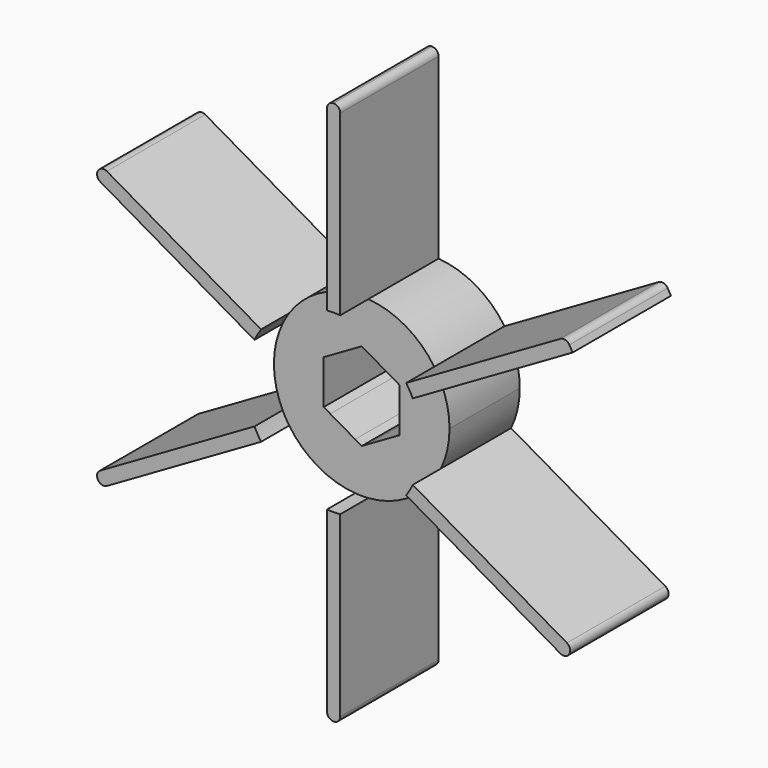
from build123d import *

# Parameters (mm, degrees)
F1_DEPTH = 10
F2_DEPTH = 14
F3_R     = 0.74999


# Not quite as in the source:
# - a fillet or chamfer is up to 0.001 mm smaller than in the source, because OpenCascade refuses the exact size
# - a feature names something its author has since deleted; it is built from what else it names


with BuildPart() as f1:
    # F0 (on Front) → F1 (new body)
    with BuildSketch(Plane.XZ):
        with BuildLine():
            ThreePointArc((9.0108627247, -4.336398616), (9.7495801768, -2.22388992), (10, 0))
            ThreePointArc((10, 0), (9.7495801768, 2.22388992), (9.0108627247, 4.336398616))
            Line((9.0108627247, 4.336398616), (4.6561359474, 1.8221959388))
            ThreePointArc((4.6561359474, 1.8221959388), (4.9132819854, 0.9271785866), (5, 0))
            ThreePointArc((5, 0), (4.9132819854, -0.9271785866), (4.6561359474, -1.8221959388))
            Line((4.6561359474, -1.8221959388), (9.0108627247, -4.336398616))
        make_face()
        with BuildLine():
            Line((4.6561359474, 1.8221959388), (9.0108627247, 4.336398616))
            ThreePointArc((9.0108627247, 4.336398616), (8.6602540378, 5), (8.2608627247, 5.6354367216))
            Line((8.2608627247, 5.6354367216), (3.9061359474, 3.1212340445))
            ThreePointArc((3.9061359474, 3.1212340445), (4.1298292758, 2.8186007438), (4.3301270189, 2.5))
            ThreePointArc((4.3301270189, 2.5), (4.5058944851, 2.1672366942), (4.6561359474, 1.8221959388))
        make_face()
        with BuildLine():
            ThreePointArc((8.2608627247, -5.6354367216), (8.6602540378, -5), (9.0108627247, -4.336398616))
            Line((9.0108627247, -4.336398616), (4.6561359474, -1.8221959388))
            ThreePointArc((4.6561359474, -1.8221959388), (4.5058944851, -2.1672366942), (4.3301270189, -2.5))
            ThreePointArc((4.3301270189, -2.5), (4.1298292758, -2.8186007438), (3.9061359474, -3.1212340445))
            Line((3.9061359474, -3.1212340445), (8.2608627247, -5.6354367216))
        make_face()
        with BuildLine():
            Line((3.9061359474, 3.1212340445), (8.2608627247, 5.6354367216))
            ThreePointArc((8.2608627247, 5.6354367216), (5, 8.6602540378), (0.75, 9.9718353376))
            Line((0.75, 9.9718353376), (0.75, 4.9434299833))
            ThreePointArc((0.75, 4.9434299833), (2.5, 4.3301270189), (3.9061359474, 3.1212340445))
        make_face()
        with BuildLine():
            Line((4.3301270189, 1.6339745962), (4.6561359474, 1.8221959388))
            ThreePointArc((4.6561359474, 1.8221959388), (4.5058944851, 2.1672366942), (4.3301270189, 2.5))
            Line((4.3301270189, 2.5), (4.3301270189, 1.6339745962))
        make_face()
        with BuildLine():
            ThreePointArc((5, 0), (4.9132819854, 0.9271785866), (4.6561359474, 1.8221959388))
            Line((4.6561359474, 1.8221959388), (4.3301270189, 1.6339745962))
            Line((4.3301270189, 1.6339745962), (4.3301270189, -1.6339745962))
            Line((4.3301270189, -1.6339745962), (4.6561359474, -1.8221959388))
            ThreePointArc((4.6561359474, -1.8221959388), (4.9132819854, -0.9271785866), (5, 0))
        make_face()
        with BuildLine():
            ThreePointArc((0.75, -9.9718353376), (5, -8.6602540378), (8.2608627247, -5.6354367216))
            Line((8.2608627247, -5.6354367216), (3.9061359474, -3.1212340445))
            ThreePointArc((3.9061359474, -3.1212340445), (2.5, -4.3301270189), (0.75, -4.9434299833))
            Line((0.75, -4.9434299833), (0.75, -9.9718353376))
        make_face()
        with BuildLine():
            ThreePointArc((4.3301270189, -2.5), (4.5058944851, -2.1672366942), (4.6561359474, -1.8221959388))
            Line((4.6561359474, -1.8221959388), (4.3301270189, -1.6339745962))
            Line((4.3301270189, -1.6339745962), (4.3301270189, -2.5))
        make_face()
        with BuildLine():
            Line((0.75, 4.9434299833), (0.75, 9.9718353376))
            ThreePointArc((0.75, 9.9718353376), (0, 10), (-0.75, 9.9718353376))
            Line((-0.75, 9.9718353376), (-0.75, 4.9434299833))
            ThreePointArc((-0.75, 4.9434299833), (-0.3760652094, 4.985837438), (0, 5))
            ThreePointArc((0, 5), (0.3760652094, 4.985837438), (0.75, 4.9434299833))
        make_face()
        with BuildLine():
            Line((3.5801270189, 2.9330127019), (3.9061359474, 3.1212340445))
            ThreePointArc((3.9061359474, 3.1212340445), (2.5, 4.3301270189), (0.75, 4.9434299833))
            Line((0.75, 4.9434299833), (0.75, 4.5669872981))
            Line((0.75, 4.5669872981), (3.5801270189, 2.9330127019))
        make_face()
        with BuildLine():
            ThreePointArc((4.3301270189, 2.5), (4.1298292758, 2.8186007438), (3.9061359474, 3.1212340445))
            Line((3.9061359474, 3.1212340445), (3.5801270189, 2.9330127019))
            Line((3.5801270189, 2.9330127019), (4.3301270189, 2.5))
        make_face()
        with BuildLine():
            ThreePointArc((-0.75, -9.9718353376), (0, -10), (0.75, -9.9718353376))
            Line((0.75, -9.9718353376), (0.75, -4.9434299833))
            ThreePointArc((0.75, -4.9434299833), (0.3760652094, -4.985837438), (0, -5))
            ThreePointArc((0, -5), (-0.3760652094, -4.985837438), (-0.75, -4.9434299833))
            Line((-0.75, -4.9434299833), (-0.75, -9.9718353376))
        make_face()
        with BuildLine():
            Line((3.5801270189, -2.9330127019), (3.9061359474, -3.1212340445))
            ThreePointArc((3.9061359474, -3.1212340445), (4.1298292758, -2.8186007438), (4.3301270189, -2.5))
            Line((4.3301270189, -2.5), (3.5801270189, -2.9330127019))
        make_face()
        with BuildLine():
            ThreePointArc((0.75, -4.9434299833), (2.5, -4.3301270189), (3.9061359474, -3.1212340445))
            Line((3.9061359474, -3.1212340445), (3.5801270189, -2.9330127019))
            Line((3.5801270189, -2.9330127019), (0.75, -4.5669872981))
            Line((0.75, -4.5669872981), (0.75, -4.9434299833))
        make_face()
        with BuildLine():
            Line((-0.75, 4.9434299833), (-0.75, 9.9718353376))
            ThreePointArc((-0.75, 9.9718353376), (-5, 8.6602540378), (-8.2608627247, 5.6354367216))
            Line((-8.2608627247, 5.6354367216), (-3.9061359474, 3.1212340445))
            ThreePointArc((-3.9061359474, 3.1212340445), (-2.5, 4.3301270189), (-0.75, 4.9434299833))
        make_face()
        with BuildLine():
            Line((0.75, 4.5669872981), (0.75, 4.9434299833))
            ThreePointArc((0.75, 4.9434299833), (0.3760652094, 4.985837438), (0, 5))
            Line((0, 5), (0.75, 4.5669872981))
        make_face()
        with BuildLine():
            ThreePointArc((-8.2608627247, -5.6354367216), (-5, -8.6602540378), (-0.75, -9.9718353376))
            Line((-0.75, -9.9718353376), (-0.75, -4.9434299833))
            ThreePointArc((-0.75, -4.9434299833), (-2.5, -4.3301270189), (-3.9061359474, -3.1212340445))
            Line((-3.9061359474, -3.1212340445), (-8.2608627247, -5.6354367216))
        make_face()
        with BuildLine():
            ThreePointArc((0, -5), (0.3760652094, -4.985837438), (0.75, -4.9434299833))
            Line((0.75, -4.9434299833), (0.75, -4.5669872981))
            Line((0.75, -4.5669872981), (0, -5))
        make_face()
        with BuildLine():
            Line((-3.9061359474, 3.1212340445), (-8.2608627247, 5.6354367216))
            ThreePointArc((-8.2608627247, 5.6354367216), (-8.6602540378, 5), (-9.0108627247, 4.336398616))
            Line((-9.0108627247, 4.336398616), (-4.6561359474, 1.8221959388))
            ThreePointArc((-4.6561359474, 1.8221959388), (-4.5058944851, 2.1672366942), (-4.3301270189, 2.5))
            ThreePointArc((-4.3301270189, 2.5), (-4.1298292758, 2.8186007438), (-3.9061359474, 3.1212340445))
        make_face()
        with BuildLine():
            Line((-0.75, 4.5669872981), (-0.75, 4.9434299833))
            ThreePointArc((-0.75, 4.9434299833), (-2.5, 4.3301270189), (-3.9061359474, 3.1212340445))
            Line((-3.9061359474, 3.1212340445), (-3.5801270189, 2.9330127019))
            Line((-3.5801270189, 2.9330127019), (-0.75, 4.5669872981))
        make_face()
        with BuildLine():
            ThreePointArc((0, 5), (-0.3760652094, 4.985837438), (-0.75, 4.9434299833))
            Line((-0.75, 4.9434299833), (-0.75, 4.5669872981))
            Line((-0.75, 4.5669872981), (0, 5))
        make_face()
        with BuildLine():
            ThreePointArc((-9.0108627247, -4.336398616), (-8.6602540378, -5), (-8.2608627247, -5.6354367216))
            Line((-8.2608627247, -5.6354367216), (-3.9061359474, -3.1212340445))
            ThreePointArc((-3.9061359474, -3.1212340445), (-4.1298292758, -2.8186007438), (-4.3301270189, -2.5))
            ThreePointArc((-4.3301270189, -2.5), (-4.5058944851, -2.1672366942), (-4.6561359474, -1.8221959388))
            Line((-4.6561359474, -1.8221959388), (-9.0108627247, -4.336398616))
        make_face()
        with BuildLine():
            Line((-0.75, -4.5669872981), (-0.75, -4.9434299833))
            ThreePointArc((-0.75, -4.9434299833), (-0.3760652094, -4.985837438), (0, -5))
            Line((0, -5), (-0.75, -4.5669872981))
        make_face()
        with BuildLine():
            ThreePointArc((-3.9061359474, -3.1212340445), (-2.5, -4.3301270189), (-0.75, -4.9434299833))
            Line((-0.75, -4.9434299833), (-0.75, -4.5669872981))
            Line((-0.75, -4.5669872981), (-3.5801270189, -2.9330127019))
            Line((-3.5801270189, -2.9330127019), (-3.9061359474, -3.1212340445))
        make_face()
        with BuildLine():
            Line((-4.6561359474, 1.8221959388), (-9.0108627247, 4.336398616))
            ThreePointArc((-9.0108627247, 4.336398616), (-10, 0), (-9.0108627247, -4.336398616))
            Line((-9.0108627247, -4.336398616), (-4.6561359474, -1.8221959388))
            ThreePointArc((-4.6561359474, -1.8221959388), (-5, 0), (-4.6561359474, 1.8221959388))
        make_face()
        with BuildLine():
            Line((-3.5801270189, 2.9330127019), (-3.9061359474, 3.1212340445))
            ThreePointArc((-3.9061359474, 3.1212340445), (-4.1298292758, 2.8186007438), (-4.3301270189, 2.5))
            Line((-4.3301270189, 2.5), (-3.5801270189, 2.9330127019))
        make_face()
        with BuildLine():
            ThreePointArc((-4.3301270189, -2.5), (-4.1298292758, -2.8186007438), (-3.9061359474, -3.1212340445))
            Line((-3.9061359474, -3.1212340445), (-3.5801270189, -2.9330127019))
            Line((-3.5801270189, -2.9330127019), (-4.3301270189, -2.5))
        make_face()
        with BuildLine():
            Line((-4.3301270189, 1.6339745962), (-4.6561359474, 1.8221959388))
            ThreePointArc((-4.6561359474, 1.8221959388), (-5, 0), (-4.6561359474, -1.8221959388))
            Line((-4.6561359474, -1.8221959388), (-4.3301270189, -1.6339745962))
            Line((-4.3301270189, -1.6339745962), (-4.3301270189, 1.6339745962))
        make_face()
        with BuildLine():
            ThreePointArc((-4.3301270189, 2.5), (-4.5058944851, 2.1672366942), (-4.6561359474, 1.8221959388))
            Line((-4.6561359474, 1.8221959388), (-4.3301270189, 1.6339745962))
            Line((-4.3301270189, 1.6339745962), (-4.3301270189, 2.5))
        make_face()
        with BuildLine():
            Line((-4.3301270189, -1.6339745962), (-4.6561359474, -1.8221959388))
            ThreePointArc((-4.6561359474, -1.8221959388), (-4.5058944851, -2.1672366942), (-4.3301270189, -2.5))
            Line((-4.3301270189, -2.5), (-4.3301270189, -1.6339745962))
        make_face()
    extrude(amount=F1_DEPTH)

    # F0 (on Front) → F2 (join)
    with BuildSketch(Plane.XZ):
        with BuildLine():
            ThreePointArc((-0.75, 9.9718353376), (0, 10), (0.75, 9.9718353376))
            Line((0.75, 9.9718353376), (0.75, 31))
            Line((0.75, 31), (-0.75, 31))
            Line((-0.75, 31), (-0.75, 9.9718353376))
        make_face()
        with BuildLine():
            Line((27.2217875173, -14.8504809472), (9.0108627247, -4.336398616))
            ThreePointArc((9.0108627247, -4.336398616), (8.6602540378, -5), (8.2608627247, -5.6354367216))
            Line((8.2608627247, -5.6354367216), (26.4717875173, -16.1495190528))
            Line((26.4717875173, -16.1495190528), (27.2217875173, -14.8504809472))
        make_face()
        with BuildLine():
            ThreePointArc((8.2608627247, 5.6354367216), (8.6602540378, 5), (9.0108627247, 4.336398616))
            Line((9.0108627247, 4.336398616), (27.2217875173, 14.8504809472))
            Line((27.2217875173, 14.8504809472), (26.4717875173, 16.1495190528))
            Line((26.4717875173, 16.1495190528), (8.2608627247, 5.6354367216))
        make_face()
        with BuildLine():
            Line((0.75, -31), (0.75, -9.9718353376))
            ThreePointArc((0.75, -9.9718353376), (0, -10), (-0.75, -9.9718353376))
            Line((-0.75, -9.9718353376), (-0.75, -31))
            Line((-0.75, -31), (0.75, -31))
        make_face()
        with BuildLine():
            Line((-26.4717875173, -16.1495190528), (-8.2608627247, -5.6354367216))
            ThreePointArc((-8.2608627247, -5.6354367216), (-8.6602540378, -5), (-9.0108627247, -4.336398616))
            Line((-9.0108627247, -4.336398616), (-27.2217875173, -14.8504809472))
            Line((-27.2217875173, -14.8504809472), (-26.4717875173, -16.1495190528))
        make_face()
        with BuildLine():
            ThreePointArc((-9.0108627247, 4.336398616), (-8.6602540378, 5), (-8.2608627247, 5.6354367216))
            Line((-8.2608627247, 5.6354367216), (-26.4717875173, 16.1495190528))
            Line((-26.4717875173, 16.1495190528), (-27.2217875173, 14.8504809472))
            Line((-27.2217875173, 14.8504809472), (-9.0108627247, 4.336398616))
        make_face()
    extrude(amount=F2_DEPTH)

    # F3 (radius 0.75 in the source; OpenCascade refuses exactly that, so slightly less here)
    f3_edges = [f1.edges().sort_by_distance(p)[0] for p in [
        (26.471788, -7, 16.149519),
        (27.221788, -7, -14.850481),
        (26.471788, -7, -16.149519),
        (0.75, -7, -31),
        (-0.75, -7, -31),
        (-26.471788, -7, -16.149519),
        (-27.221788, -7, -14.850481),
        (-26.471788, -7, 16.149519),
        (-27.221788, -7, 14.850481),
        (0.75, -7, 31),
        (-0.75, -7, 31),
    ]]
    fillet(f3_edges, radius=F3_R)


solid = f1.part
